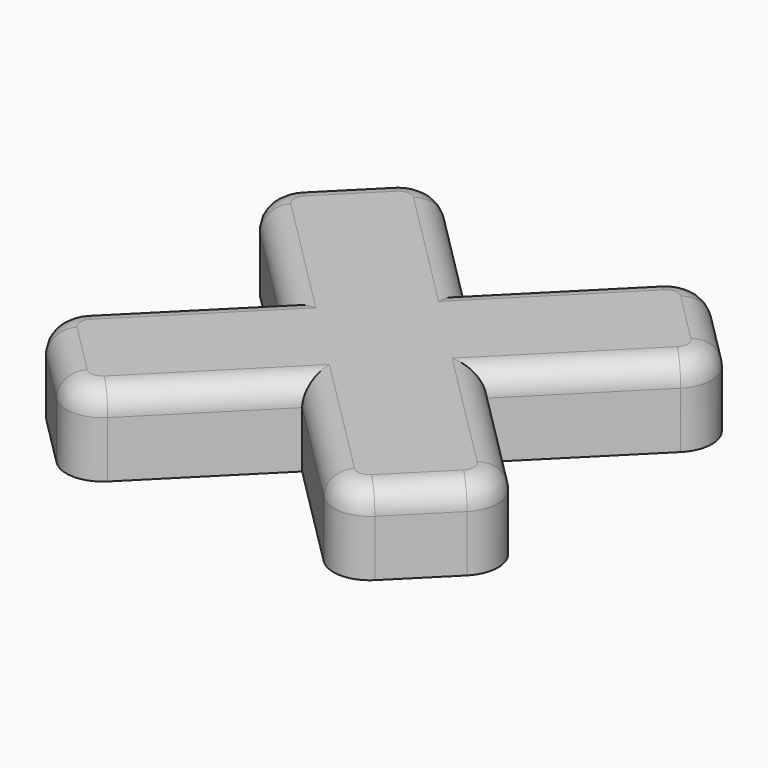
from build123d import *

# Parameters (mm, degrees)
F1_DEPTH     = 10
F2_DEPTH     = 8
F3_R         = 3
F4_T1_DEPTH  = 21.25
F4_T4_ANGLE  = 90
F4_T6_ANGLE  = 90
F4_T8_ANGLE  = 90
F4_T10_ANGLE = 90
F4_T12_ANGLE = 90
F4_T14_ANGLE = 90
F4_T16_ANGLE = 90
F4_T18_ANGLE = 90


# Not quite as in the source:
# - a fillet or chamfer that OpenCascade refuses, or shapes differently, is made with other operations: its cross-section is extruded or revolved along the edge and cut away or added


with BuildPart() as f1:
    # F0 (on Top) → F1 (new body)
    with BuildSketch(Plane.XY):
        Polygon((25.7107810123, -8.5209181738), (27.2851523571, -8.9427697042), (27.7070038876, -10.5171410491), (33.0728534806, -15.8829906421), (49.6898628385, 0.7340187158), (36.9619407771, 13.4619407771), (20.3449314192, -3.1550685808), align=None)
        Polygon((33.0728534806, -15.8829906421), (27.7070038876, -10.5171410491), (29.8254495283, -18.4232878133), (22.8852285904, -25.3635087511), (14.9790818262, -23.2450631104), (20.3449314192, -28.6109127035), align=None)
        Polygon((17.8046342481, -6.4024725331), (25.7107810123, -8.5209181738), (20.3449314192, -3.1550685808), (7.6170093579, -15.8829906421), (12.9828589509, -21.2488402351), (10.8644133102, -13.342693471), align=None)
        Polygon((49.6898628385, -32.5), (33.0728534806, -15.8829906421), (20.3449314192, -28.6109127035), (36.9619407771, -45.2279220614), align=None)
        Polygon((7.6170093579, -15.8829906421), (20.3449314192, -3.1550685808), (3.7279220614, 13.4619407771), (-9, 0.7340187158), align=None)
        Polygon((3.7279220614, -45.2279220614), (20.3449314192, -28.6109127035), (14.9790818262, -23.2450631104), (13.4047104814, -22.82321158), (12.9828589509, -21.2488402351), (7.6170093579, -15.8829906421), (-9, -32.5), align=None)
        Polygon((29.8254495283, -18.4232878133), (27.7070038876, -10.5171410491), (25.7107810123, -8.5209181738), (17.8046342481, -6.4024725331), (10.8644133102, -13.342693471), (12.9828589509, -21.2488402351), (14.9790818262, -23.2450631104), (22.8852285904, -25.3635087511), align=None)
        Polygon((27.7070038876, -10.5171410491), (27.2851523571, -8.9427697042), (25.7107810123, -8.5209181738), align=None)
        Polygon((13.4047104814, -22.82321158), (14.9790818262, -23.2450631104), (12.9828589509, -21.2488402351), align=None)
    extrude(amount=F1_DEPTH)

    # F0 (on Top) → F2 (cut)
    with BuildSketch(Plane.XY):
        Polygon((29.8254495283, -18.4232878133), (27.7070038876, -10.5171410491), (25.7107810123, -8.5209181738), (17.8046342481, -6.4024725331), (10.8644133102, -13.342693471), (12.9828589509, -21.2488402351), (14.9790818262, -23.2450631104), (22.8852285904, -25.3635087511), align=None)
        Polygon((13.4047104814, -22.82321158), (14.9790818262, -23.2450631104), (12.9828589509, -21.2488402351), align=None)
        Polygon((27.7070038876, -10.5171410491), (27.2851523571, -8.9427697042), (25.7107810123, -8.5209181738), align=None)
    extrude(amount=F2_DEPTH, mode=Mode.SUBTRACT)

    # F3
    f3_edges = [f1.edges().sort_by_distance(p)[0] for p in [
        (43.325902, 7.09798, 10),
        (28.653436, 5.153436, 10),
        (12.036427, 5.153436, 10),
        (-2.636039, 7.09798, 10),
        (-0.691495, -7.574486, 10),
        (-0.691495, -24.191495, 10),
        (-2.636039, -38.863961, 10),
        (12.036427, -36.919417, 10),
        (28.653436, -36.919417, 10),
        (43.325902, -38.863961, 10),
        (41.381358, -24.191495, 10),
        (41.381358, -7.574486, 10),
    ]]
    fillet(f3_edges, radius=F3_R)

    # F4: fillet of radius 4.5 on 8 edges, made by hand

    # F4_s2 → F4_t1 (cut)
    with BuildSketch(Plane.XY.offset(-11.25)):
        with BuildLine():
            ThreePointArc((40.1439212925, 10.2799602618), (36.9619407771, 11.5979797464), (33.7799602618, 10.2799602618))
            Line((33.7799602618, 10.2799602618), (36.9619407771, 13.4619407771))
            Line((36.9619407771, 13.4619407771), (40.1439212925, 10.2799602618))
        make_face()
        with BuildLine():
            ThreePointArc((46.5078823231, 3.9159992311), (47.8259018078, 0.7340187158), (46.5078823231, -2.4479617996))
            Line((46.5078823231, -2.4479617996), (49.6898628385, 0.7340187158))
            Line((49.6898628385, 0.7340187158), (46.5078823231, 3.9159992311))
        make_face()
        with BuildLine():
            ThreePointArc((46.5078823231, -29.3180194847), (47.8259018078, -32.5), (46.5078823231, -35.6819805153))
            Line((46.5078823231, -35.6819805153), (49.6898628385, -32.5))
            Line((49.6898628385, -32.5), (46.5078823231, -29.3180194847))
        make_face()
        with BuildLine():
            ThreePointArc((40.1439212925, -42.045941546), (36.9619407771, -43.3639610307), (33.7799602618, -42.045941546))
            Line((33.7799602618, -42.045941546), (36.9619407771, -45.2279220614))
            Line((36.9619407771, -45.2279220614), (40.1439212925, -42.045941546))
        make_face()
        with BuildLine():
            ThreePointArc((6.9099025767, -42.045941546), (3.7279220614, -43.3639610307), (0.545941546, -42.045941546))
            Line((0.545941546, -42.045941546), (3.7279220614, -45.2279220614))
            Line((3.7279220614, -45.2279220614), (6.9099025767, -42.045941546))
        make_face()
        with BuildLine():
            ThreePointArc((-5.8180194847, -29.3180194847), (-7.1360389693, -32.5), (-5.8180194847, -35.6819805153))
            Line((-5.8180194847, -35.6819805153), (-9, -32.5))
            Line((-9, -32.5), (-5.8180194847, -29.3180194847))
        make_face()
        with BuildLine():
            ThreePointArc((-5.8180194847, 3.9159992311), (-7.1360389693, 0.7340187158), (-5.8180194847, -2.4479617996))
            Line((-5.8180194847, -2.4479617996), (-9, 0.7340187158))
            Line((-9, 0.7340187158), (-5.8180194847, 3.9159992311))
        make_face()
        with BuildLine():
            ThreePointArc((6.9099025767, 10.2799602618), (3.7279220614, 11.5979797464), (0.545941546, 10.2799602618))
            Line((0.545941546, 10.2799602618), (3.7279220614, 13.4619407771))
            Line((3.7279220614, 13.4619407771), (6.9099025767, 10.2799602618))
        make_face()
    extrude(amount=F4_T1_DEPTH, mode=Mode.SUBTRACT)

    # F4_s3 → F4_t4 (revolve, cut)
    with BuildSketch(Plane(origin=(-1.6850288425, 1.6850288425, 0), x_dir=(0, 0, 1), z_dir=(0.7071067812, -0.7071067812, 0))):
        with BuildLine():
            ThreePointArc((10, -9.1550685808), (9.1213203436, -11.2763889243), (7, -12.1550685808))
            Line((7, -12.1550685808), (10, -12.1550685808))
            Line((10, -12.1550685808), (10, -9.1550685808))
        make_face()
    revolve(axis=Axis((3.7279220614, 7.0979797464, 10), (0, 0, 1)), revolution_arc=F4_T4_ANGLE, mode=Mode.SUBTRACT)

    # F4_s5 → F4_t6 (revolve, cut)
    with BuildSketch(Plane(origin=(-0.9510101268, -0.9510101268, 0), x_dir=(0, 0, 1), z_dir=(0.7071067812, 0.7071067812, 0))):
        with BuildLine():
            ThreePointArc((10, -3.8829906421), (9.1213203436, -6.0043109857), (7, -6.8829906421))
            Line((7, -6.8829906421), (10, -6.8829906421))
            Line((10, -6.8829906421), (10, -3.8829906421))
        make_face()
    revolve(axis=Axis((-2.6360389693, 0.7340187158, 10), (0, 0, 1)), revolution_arc=F4_T6_ANGLE, mode=Mode.SUBTRACT)

    # F4_s7 → F4_t8 (revolve, cut)
    with BuildSketch(Plane(origin=(-17.5680194847, -17.5680194847, 0), x_dir=(0, 0, 1), z_dir=(0.7071067812, 0.7071067812, 0))):
        with BuildLine():
            ThreePointArc((10, 19.6170093579), (9.1213203436, 17.4956890143), (7, 16.6170093579))
            Line((7, 16.6170093579), (10, 16.6170093579))
            Line((10, 16.6170093579), (10, 19.6170093579))
        make_face()
    revolve(axis=Axis((-2.6360389693, -32.5, 10), (0, 0, 1)), revolution_arc=F4_T8_ANGLE, mode=Mode.SUBTRACT)

    # F4_s9 → F4_t10 (revolve, cut)
    with BuildSketch(Plane(origin=(21.295941546, -21.295941546, 0), x_dir=(0, 0, 1), z_dir=(-0.7071067812, 0.7071067812, 0))):
        with BuildLine():
            ThreePointArc((10, -26.3449314192), (9.1213203436, -28.4662517628), (7, -29.3449314192))
            Line((7, -29.3449314192), (10, -29.3449314192))
            Line((10, -29.3449314192), (10, -26.3449314192))
        make_face()
    revolve(axis=Axis((3.7279220614, -38.8639610307, 10), (0, 0, 1)), revolution_arc=F4_T10_ANGLE, mode=Mode.SUBTRACT)

    # F4_s11 → F4_t12 (revolve, cut)
    with BuildSketch(Plane(origin=(37.9129509039, -37.9129509039, 0), x_dir=(0, 0, 1), z_dir=(-0.7071067812, 0.7071067812, 0))):
        with BuildLine():
            ThreePointArc((10, -2.8449314192), (9.1213203436, -4.9662517628), (7, -5.8449314192))
            Line((7, -5.8449314192), (10, -5.8449314192))
            Line((10, -5.8449314192), (10, -2.8449314192))
        make_face()
    revolve(axis=Axis((36.9619407771, -38.8639610307, 10), (0, 0, 1)), revolution_arc=F4_T12_ANGLE, mode=Mode.SUBTRACT)

    # F4_s13 → F4_t14 (revolve, cut)
    with BuildSketch(Plane(origin=(5.4129509039, 5.4129509039, 0), x_dir=(0, 0, 1), z_dir=(-0.7071067812, -0.7071067812, 0))):
        with BuildLine():
            ThreePointArc((10, -55.1170093579), (9.1213203436, -57.2383297014), (7, -58.1170093579))
            Line((7, -58.1170093579), (10, -58.1170093579))
            Line((10, -58.1170093579), (10, -55.1170093579))
        make_face()
    revolve(axis=Axis((43.3259018078, -32.5, 10), (0, 0, 1)), revolution_arc=F4_T14_ANGLE, mode=Mode.SUBTRACT)

    # F4_s15 → F4_t16 (revolve, cut)
    with BuildSketch(Plane(origin=(22.0299602618, 22.0299602618, 0), x_dir=(0, 0, 1), z_dir=(-0.7071067812, -0.7071067812, 0))):
        with BuildLine():
            ThreePointArc((10, -31.6170093579), (9.1213203436, -33.7383297014), (7, -34.6170093579))
            Line((7, -34.6170093579), (10, -34.6170093579))
            Line((10, -34.6170093579), (10, -31.6170093579))
        make_face()
    revolve(axis=Axis((43.3259018078, 0.7340187158, 10), (0, 0, 1)), revolution_arc=F4_T16_ANGLE, mode=Mode.SUBTRACT)

    # F4_s17 → F4_t18 (revolve, cut)
    with BuildSketch(Plane(origin=(14.9319805153, -14.9319805153, 0), x_dir=(0, 0, 1), z_dir=(0.7071067812, -0.7071067812, 0))):
        with BuildLine():
            ThreePointArc((10, -32.6550685808), (9.1213203436, -34.7763889243), (7, -35.6550685808))
            Line((7, -35.6550685808), (10, -35.6550685808))
            Line((10, -35.6550685808), (10, -32.6550685808))
        make_face()
    revolve(axis=Axis((36.9619407771, 7.0979797464, 10), (0, 0, 1)), revolution_arc=F4_T18_ANGLE, mode=Mode.SUBTRACT)


solid = f1.part
